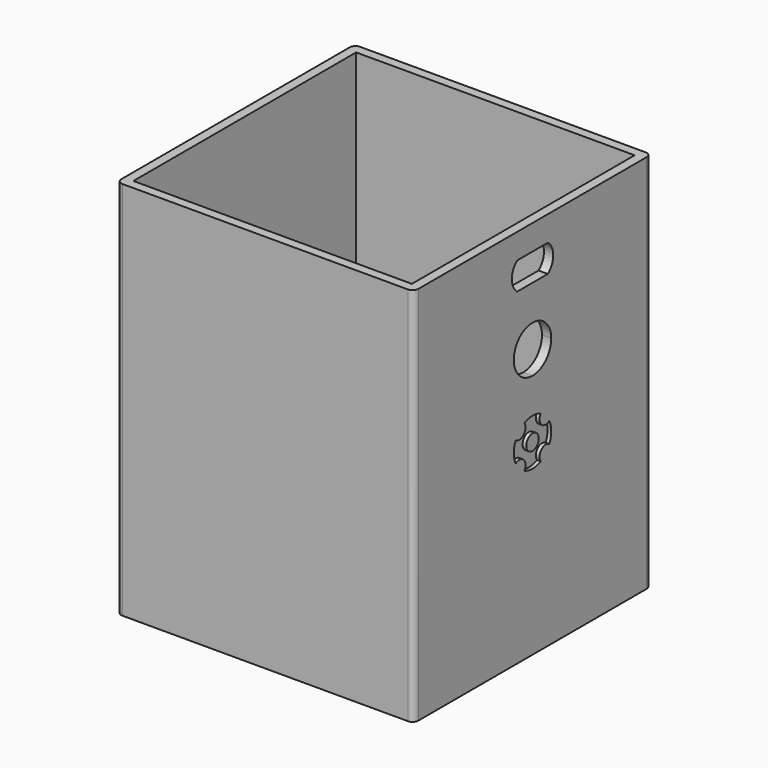
from build123d import *

# Parameters (mm, degrees)
F0_W     = 101.6
F0_H     = 101.6
F0_W_2   = 95.25
F0_H_2   = 95.25
F1_DEPTH = 130
F2_R     = 2
F3_W     = 6.54
F3_H     = 9.4
F4_DEPTH = 3.175
F5_R     = 2.6666666667
F6_DEPTH = 1.27


# Not quite as in the source:
# - a length typed as a fraction of an inch, garbled in the dataset ("3 / 203.2 mm" for 3/8 in), is restored


with BuildPart() as f1:
    # F0 (on Top) → F1 (new body)
    with BuildSketch(Plane.XY):
        Rectangle(F0_W, F0_H)
        Rectangle(F0_W_2, F0_H_2, mode=Mode.SUBTRACT)
    extrude(amount=F1_DEPTH)

    # F2
    f2_edges = [f1.edges().sort_by_distance(p)[0] for p in [
        (50.8, 50.8, 65),
        (-50.8, 50.8, 65),
        (50.8, -50.8, 65),
        (-50.8, -50.8, 65),
    ]]
    fillet(f2_edges, radius=F2_R)

    # F3 (on face) → F4 (cut)
    with BuildSketch(Plane.YZ.offset(50.8)):
        with Locations((-3.27, 116.7)):
            Rectangle(F3_W, F3_H)
        with BuildLine():
            Line((-6.54, 112), (-6.54, 121.4))
            ThreePointArc((-6.54, 121.4), (-8.85, 116.7), (-6.54, 112))
        make_face()
        with Locations((3.27, 116.7)):
            Rectangle(F3_W, F3_H)
        with BuildLine():
            ThreePointArc((6.54, 112), (8.85, 116.7), (6.54, 121.4))
            Line((6.54, 121.4), (6.54, 112))
        make_face()
        with BuildLine():
            Line((0, 84), (0, 100))
            ThreePointArc((0, 100), (-8, 92), (0, 84))
        make_face()
        with BuildLine():
            ThreePointArc((8, 92), (5.6568542495, 97.6568542495), (0, 100))
            Line((0, 100), (0, 84))
            ThreePointArc((0, 84), (5.6568542495, 86.3431457505), (8, 92))
        make_face()
    extrude(amount=-F4_DEPTH, mode=Mode.SUBTRACT)

    # F5 (on face) → F6 (cut)
    with BuildSketch(Plane.YZ.offset(50.8)):
        with BuildLine():
            Line((0, 84), (0, 100))
            ThreePointArc((0, 100), (-8, 92), (0, 84))
        make_face()
        with BuildLine():
            ThreePointArc((8, 92), (5.6568542495, 97.6568542495), (0, 100))
            Line((0, 100), (0, 84))
            ThreePointArc((0, 84), (5.6568542495, 86.3431457505), (8, 92))
        make_face()
        with BuildLine():
            ThreePointArc((-3.4833400656, 71.2018290724), (-3.7712361663, 67.7712361663), (-7.2018290724, 67.4833400656))
            ThreePointArc((-7.2018290724, 67.4833400656), (-8, 64), (-7.2018290724, 60.5166599344))
            ThreePointArc((-7.2018290724, 60.5166599344), (-3.7712361663, 60.2287638337), (-3.4833400656, 56.7981709276))
            ThreePointArc((-3.4833400656, 56.7981709276), (0, 56), (3.4833400656, 56.7981709276))
            ThreePointArc((3.4833400656, 56.7981709276), (3.7712361663, 60.2287638337), (7.2018290724, 60.5166599344))
            ThreePointArc((7.2018290724, 60.5166599344), (8, 64), (7.2018290724, 67.4833400656))
            ThreePointArc((7.2018290724, 67.4833400656), (3.7712361663, 67.7712361663), (3.4833400656, 71.2018290724))
            ThreePointArc((3.4833400656, 71.2018290724), (0, 72), (-3.4833400656, 71.2018290724))
        make_face()
        with Locations((0, 64)):
            Circle(F5_R, mode=Mode.SUBTRACT)
    extrude(amount=-F6_DEPTH, mode=Mode.SUBTRACT)


solid = f1.part
